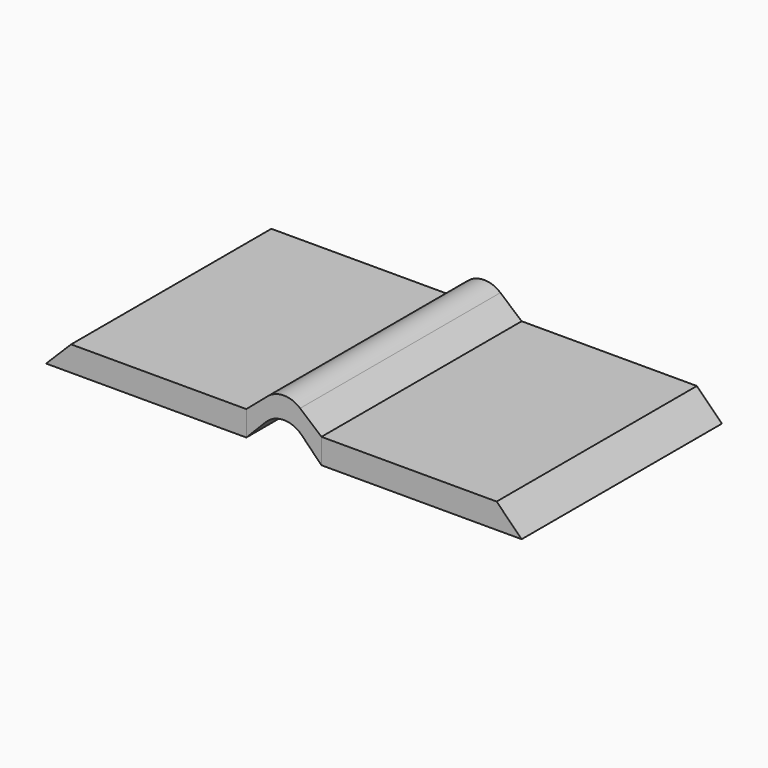
from build123d import *

# Parameters (mm, degrees)
F0_W      = 8
F0_H      = 10
F1_DEPTH  = 1
F3_DEPTH  = 10
F4_R      = 1
F5_SIZE   = 0.99999
F5_2_SIZE = 0.99999


# Not quite as in the source:
# - a fillet or chamfer is up to 0.001 mm smaller than in the source, because OpenCascade refuses the exact size


with BuildPart() as f1:
    # F0 (on Top) → F1 (new body)
    with BuildSketch(Plane.XY):
        with Locations((12.0103892572, -3.1608146429)):
            Rectangle(F0_W, F0_H)
    extrude(amount=F1_DEPTH)

    # F5#2 (size 1 in the source; OpenCascade refuses exactly that, so slightly less here)
    f5_2_edges = [f1.edges().sort_by_distance(p)[0] for p in [
        (16.010389, -3.160815, 1),
    ]]
    chamfer(f5_2_edges, length=F5_2_SIZE)


with BuildPart() as f1b:
    # F0 (on Top) → F1, piece 2 (new body)
    with BuildSketch(Plane.XY):
        with Locations((1.0103892572, -3.1608146429)):
            Rectangle(F0_W, F0_H)
    extrude(amount=F1_DEPTH)

    # F5 (size 1 in the source; OpenCascade refuses exactly that, so slightly less here)
    f5_edges = [f1b.edges().sort_by_distance(p)[0] for p in [
        (-2.989611, -3.160815, 1),
    ]]
    chamfer(f5_edges, length=F5_SIZE)


with BuildPart() as f3:
    # F2 (on face) → F3 (new body, through all)
    with BuildSketch(Plane(origin=(0, 1.8391853571, 0), x_dir=(-1, 0, 0), z_dir=(0, 1, 0))):
        Polygon((-6.5103892572, 2.2825093409), (-8.0103892572, 1), (-8.0103892572, 0), (-6.5103892572, 1.5325093409), (-5.0103892572, 0), (-5.0103892572, 1), align=None)
    extrude(amount=-F3_DEPTH)

    # F4
    f4_edges = [f3.edges().sort_by_distance(p)[0] for p in [
        (6.510389, -3.160815, 1.532509),
        (6.510389, -3.160815, 2.282509),
    ]]
    fillet(f4_edges, radius=F4_R)


solid = Compound([f1.part, f1b.part, f3.part])
